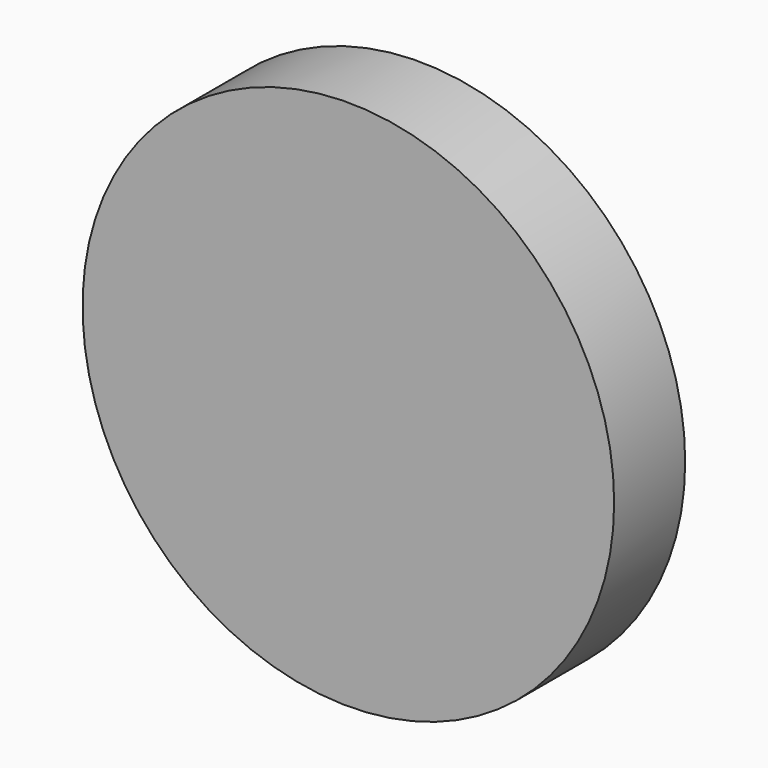
from build123d import *

# Parameters (mm, degrees)
F0_R     = 76.0405543096
F1_DEPTH = 25.4


# Not quite as in the source:
# - the program builds the solid bodies; features that only make, move or delete a surface that nothing else refers to are left out


with BuildPart() as f1:
    # F0 (on Front) → F1 (new body)
    with BuildSketch(Plane.XZ):
        Circle(F0_R)
    extrude(amount=F1_DEPTH)


solid = f1.part
